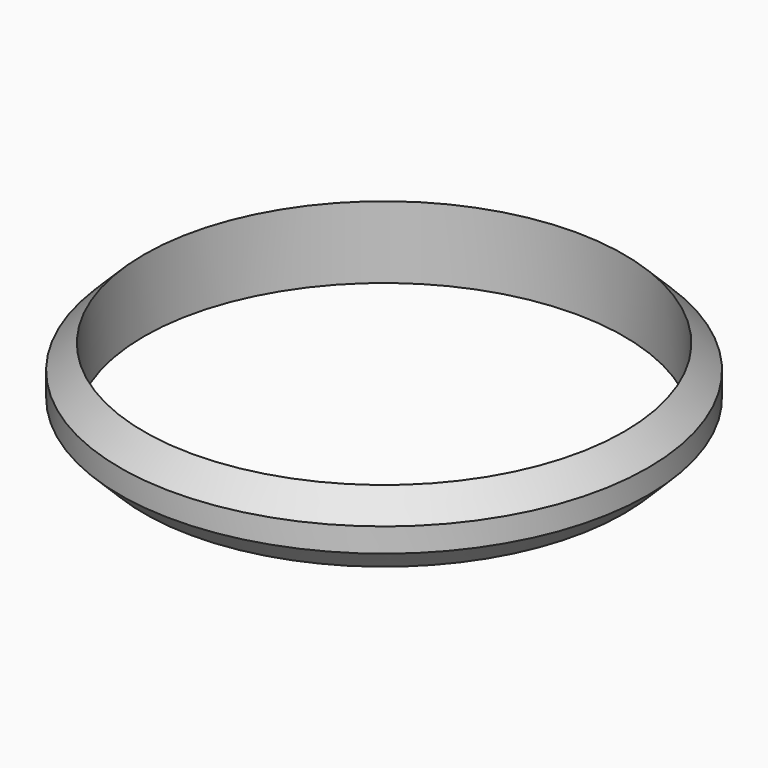
from build123d import *

# Parameters (mm, degrees)
F0_R     = 11
F1_DEPTH = 3
F2_R     = 10
F3_DEPTH = 3
F4_SIZE  = 0.99999


# Not quite as in the source:
# - a fillet or chamfer is up to 0.001 mm smaller than in the source, because OpenCascade refuses the exact size


with BuildPart() as f1:
    # F0 (on Top) → F1 (new body)
    with BuildSketch(Plane.XY):
        Circle(F0_R)
    extrude(amount=F1_DEPTH)

    # F2 (on face) → F3 (cut)
    with BuildSketch(Plane.XY.offset(3)):
        Circle(F2_R)
    extrude(amount=-F3_DEPTH, mode=Mode.SUBTRACT)

    # F4 (size 1 in the source; OpenCascade refuses exactly that, so slightly less here)
    f4_edges = [f1.edges().sort_by_distance(p)[0] for p in [
        (-11, 0, 3),
        (-11, 0, 0),
    ]]
    chamfer(f4_edges, length=F4_SIZE)


solid = f1.part
